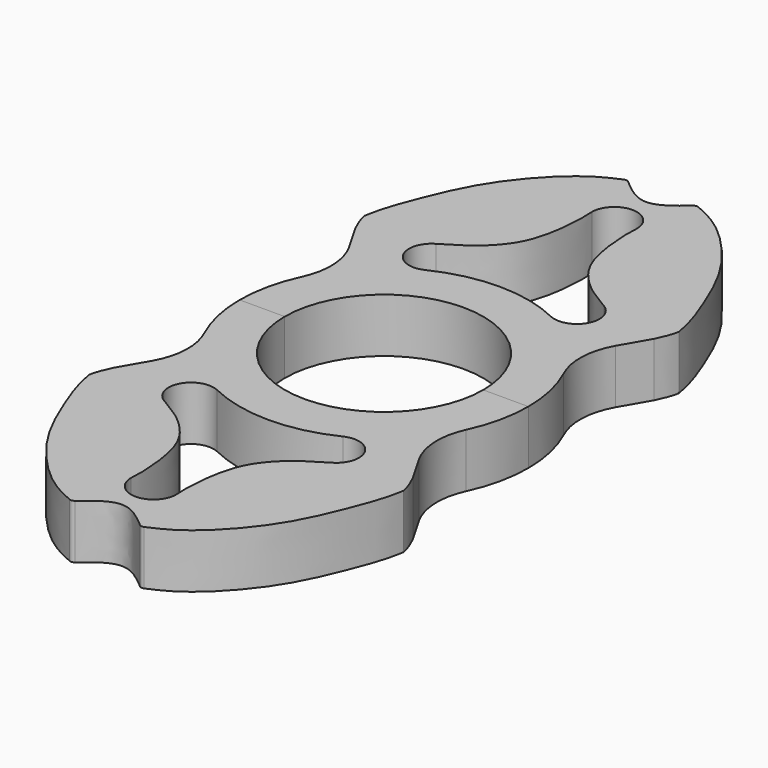
from build123d import *
from build123d import SkipClean  # not in build123d's __all__

# Parameters (mm, degrees)
F1_DEPTH = 6


with BuildPart() as f1:
    # F0 (on Top) → F1 (new body)
    with BuildSketch(Plane.XY):
        with BuildLine():
            Line((11, 0), (16, 1.6e-09))
            ThreePointArc((16, 1.6e-09), (15.6213478003, 3.4602735298), (14.5033133881, 6.7567670352))
            ThreePointArc((14.5033133881, 6.7567670352), (13.8069409235, 10.2032214588), (14.7578233989, 13.5883071625))
            Line((14.7578233989, 13.5883071625), (16.5472631726, 16.6890034893))
            add(Edge.make_bspline(
                [(16.5472631726, 16.6890034893), (16.9038641607, 17.448339213), (17.2604651496, 18.2076749358), (17.4132885774, 19.0774979941)],
                knots=[0, 0, 0, 0, 0.470604118, 0.470604118, 0.470604118, 0.470604118], degree=3))
            add(Edge.make_bspline(
                [(17.4132885774, 19.0774979941), (17.1601349358, 20.8732534921), (15.5298067403, 25.2595570374), (12.9266999076, 31.0960374776), (8.0354918433, 36.4833822131), (5.4328634191, 37.8317600488), (4.1245531765, 38.3842009986)],
                knots=[0.1468390725, 0.1468390725, 0.1468390725, 0.1468390725, 0.3630340887, 0.5865738983, 0.817044302, 0.9876810607, 0.9876810607, 0.9876810607, 0.9876810607], degree=3))
            ThreePointArc((4.1245531765, 38.3842009986), (3.8530941398, 38.4176233235), (3.6046637333, 38.3032144361))
            add(Edge.make_bspline(
                [(-3.6046637371, 38.3032144358), (-2.4031091586, 37.2733390488), (-1.8e-09, 35.3316097761), (2.4031091549, 37.2733390491), (3.6046637333, 38.3032144361)],
                knots=[0.030390823, 0.030390823, 0.030390823, 0.030390823, 0.5, 0.969609177, 0.969609177, 0.969609177, 0.969609177], degree=3))
            ThreePointArc((-3.6046637371, 38.3032144358), (-3.8530941436, 38.4176233231), (-4.1245531803, 38.3842009982))
            add(Edge.make_bspline(
                [(-17.4132885793, 19.0774979924), (-17.1601349379, 20.8732534904), (-15.5298067428, 25.2595570358), (-12.9266999107, 31.0960374763), (-8.035491847, 36.4833822123), (-5.4328634228, 37.8317600483), (-4.1245531803, 38.3842009982)],
                knots=[0.1468390725, 0.1468390725, 0.1468390725, 0.1468390725, 0.3630340887, 0.5865738983, 0.817044302, 0.9876810607, 0.9876810607, 0.9876810607, 0.9876810607], degree=3))
            add(Edge.make_bspline(
                [(-16.5472631742, 16.6890034877), (-16.9038641624, 17.4483392113), (-17.2604651514, 18.2076749341), (-17.4132885793, 19.0774979924)],
                knots=[0, 0, 0, 0, 0.470604118, 0.470604118, 0.470604118, 0.470604118], degree=3))
            Line((-16.5472631742, 16.6890034877), (-14.8065510117, 13.6740015815))
            ThreePointArc((-14.8065510117, 13.6740015815), (-14.7820464093, 13.6312344311), (-14.7578234003, 13.588307161))
            ThreePointArc((-14.7578234003, 13.588307161), (-13.8069409246, 10.2032214574), (-14.5033133887, 6.7567670338))
            ThreePointArc((-14.5033133887, 6.7567670338), (-15.6213478009, 3.4602735275), (-16, -1.6e-09))
            Line((-16, -1.6e-09), (-11, 0))
            ThreePointArc((-11, 0), (0, 11), (11, 0))
        make_face()
        with BuildLine():
            ThreePointArc((-2.5000000016, 31.9088473916), (-1.7e-09, 34.4088473916), (2.4999999984, 31.9088473919))
            add(Edge.make_bspline(
                [(2.4999999984, 31.9088473919), (2.4331220875, 30.6490394366), (2.4535157786, 30.0127263528), (2.8986373447, 23.7894092906), (6.9226723249, 20.184951896), (7.2970524431, 20.0978087895), (9.3067939385, 18.8178154741)],
                knots=[0, 0, 0, 0, 0.1919590959, 0.4953854958, 0.7661719362, 1, 1, 1, 1], degree=3))
            ThreePointArc((9.3067939385, 18.8178154741), (10.256799547, 15.4836064731), (6.9615764648, 14.4061255418))
            ThreePointArc((6.9615764648, 14.4061255418), (-8e-10, 16), (-6.9615764662, 14.4061255411))
            ThreePointArc((-6.9615764662, 14.4061255411), (-10.2567995485, 15.483606472), (-9.3067939404, 18.8178154732))
            add(Edge.make_bspline(
                [(-2.5000000016, 31.9088473916), (-2.4331220905, 30.6490394363), (-2.4535157816, 30.0127263526), (-2.898637347, 23.7894092903), (-6.9226723269, 20.1849518953), (-7.2970524451, 20.0978087888), (-9.3067939404, 18.8178154732)],
                knots=[0, 0, 0, 0, 0.1919590959, 0.4953854958, 0.7661719362, 1, 1, 1, 1], degree=3))
        make_face(mode=Mode.SUBTRACT)
    extrude(amount=F1_DEPTH)

    # F2: F1 across plane


with BuildPart() as f1_1:
    add(f1.part, clean=False)
    with SkipClean():  # cleaning this boolean's faces spoils the solid; the shape is the same uncleaned
        add(f1.part.mirror(Plane.XZ), clean=False)


solid = f1_1.part
